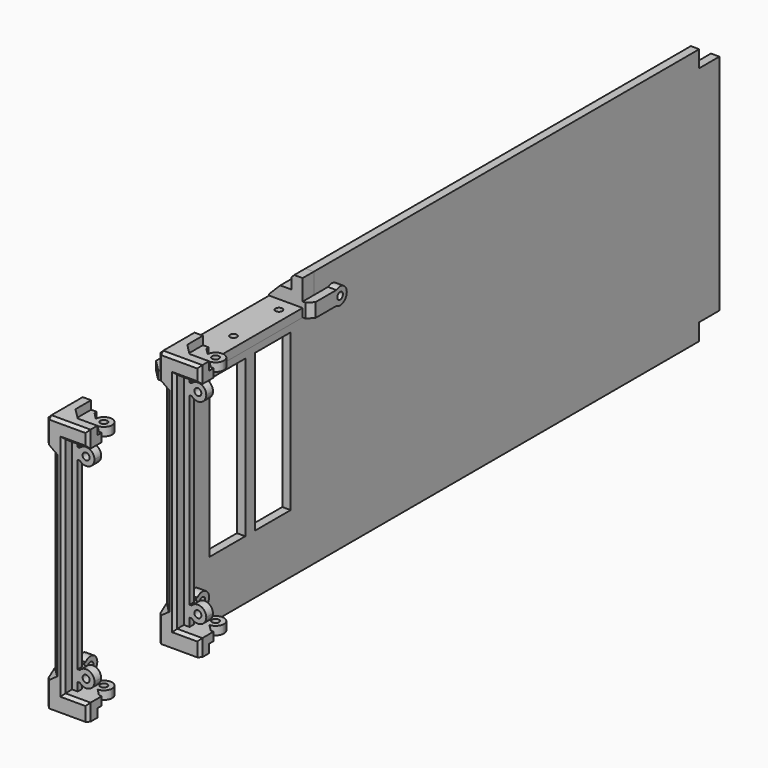
from build123d import *

# Parameters (mm, degrees)
F1_DEPTH     = 6
F2_W         = 2
F2_H         = 2
F3_DEPTH     = 5
F5_DEPTH     = 35
F7_DEPTH     = 3
F8_R         = 1.25
F9_DEPTH     = 3
F11_DEPTH    = 4
F13_DEPTH    = 3
F15_DEPTH    = 3
F17_SIZE     = 0.99999
F18_SIZE     = 2
F20_W        = 7.1945152003
F20_H        = 11.8572201729
F21_DEPTH    = 25
F23_W        = 10
F23_H        = 5
F24_DEPTH    = 4
F25_W        = 5
F25_H        = 4.5
F25_W_2      = 3
F25_W_3      = 7
F25_H_2      = 3
F26_DEPTH    = 8
F27_SIZE     = 4
F28_SIZE     = 3
F29_R        = 1.25
F30_DEPTH    = 3
F31_W        = 5
F31_H        = 5
F32_DEPTH    = 3
F33_SIZE     = 2
F34_T1_DEPTH = 3.071682988
F34_T3_DEPTH = 10.1433659759
F34_T5_DEPTH = 7.471682988
F36_DEPTH    = 3
F22_W        = 7.95
F22_H        = 56
F22_W_2      = 15.9
F37_DEPTH    = 25


# Not quite as in the source:
# - a fillet or chamfer that OpenCascade refuses, or shapes differently, is made with other operations: its cross-section is extruded or revolved along the edge and cut away or added
# - a fillet or chamfer is up to 0.001 mm smaller than in the source, because OpenCascade refuses the exact size
# - a feature names something its author has since deleted; it is built from what else it names


with BuildPart() as f1:
    # F0 (on Top) → F1 (new body)
    with BuildSketch(Plane.XY):
        Polygon((-29.7051688433, 8.7922193985), (-30.7051688433, 8.7922193985), (-30.7051688433, -6.2077806015), (-15.7051688433, -6.2077806015), (-15.7051688433, -5.2077806015), (-15.7051688433, -0.2077806015), (-24.7051688433, -0.2077806015), (-24.7051688433, 8.7922193985), align=None)
    extrude(amount=F1_DEPTH)

    # F2 (on face) → F3 (join)
    with BuildSketch(Plane.XY.offset(6)):
        with Locations((-23.7051688433, -1.2077806015)):
            Rectangle(F2_W, F2_H)
        Polygon((-26.7051688433, -0.2077806015), (-30.7051688433, -0.2077806015), (-30.7051688433, -5.2077806015), (-29.7051688433, -6.2077806015), (-24.7051688433, -6.2077806015), (-24.7051688433, -2.2077806015), (-24.7051688433, -0.2077806015), align=None)
        with Locations((-25.7051688433, 0.7922193985)):
            Rectangle(F2_W, F2_H)
    extrude(amount=F3_DEPTH)

    # F4 (on face) → F5 (join)
    with BuildSketch(Plane.XY.offset(11)):
        Polygon((-26.7051688433, -6.2077806015), (-24.7051688433, -6.2077806015), (-24.7051688433, -2.2077806015), (-22.7051688433, -2.2077806015), (-22.7051688433, -0.2077806015), (-24.7051688433, -0.2077806015), (-24.7051688433, 1.7922193985), (-26.7051688433, 1.7922193985), (-26.7051688433, -0.2077806015), (-30.7051688433, -0.2077806015), (-30.7051688433, -2.2077806015), align=None)
    extrude(amount=F5_DEPTH)

    # F6 (on face) → F7 (join)
    with BuildSketch(Plane.XZ.offset(2.2077806015)):
        with BuildLine():
            ThreePointArc((-21.9412368208, 13), (-22.5076859202, 12.0704662693), (-22.7051688433, 11))
            ThreePointArc((-22.7051688433, 11), (-22.5076859202, 9.9295337307), (-21.9412368208, 9))
            ThreePointArc((-21.9412368208, 9), (-18.634702574, 8.1974829231), (-16.7051688433, 11))
            ThreePointArc((-16.7051688433, 11), (-18.634702574, 13.8025170769), (-21.9412368208, 13))
        make_face()
        with BuildLine():
            ThreePointArc((-18.4551688433, 11), (-19.7051688433, 9.75), (-20.9551688433, 11))
            ThreePointArc((-20.9551688433, 11), (-19.7051688433, 12.25), (-18.4551688433, 11))
        make_face(mode=Mode.SUBTRACT)
        with BuildLine():
            Line((-22.7051688433, 13), (-22.7051688433, 11))
            ThreePointArc((-22.7051688433, 11), (-22.5076859202, 12.0704662693), (-21.9412368208, 13))
            Line((-21.9412368208, 13), (-22.7051688433, 13))
        make_face()
        with BuildLine():
            Line((-22.7051688433, 11), (-22.7051688433, 9))
            Line((-22.7051688433, 9), (-21.9412368208, 9))
            ThreePointArc((-21.9412368208, 9), (-22.5076859202, 9.9295337307), (-22.7051688433, 11))
        make_face()
    extrude(amount=-F7_DEPTH)

    # F8 (on face) → F9 (join)
    with BuildSketch(Plane(origin=(-26.7051688433, 0, 0), x_dir=(0, -1, 0), z_dir=(-1, 0, 0))):
        with BuildLine():
            Line((-2.556151421, 9), (-1.7922193985, 9))
            Line((-1.7922193985, 9), (-1.7922193985, 11))
            ThreePointArc((-1.7922193985, 11), (-1.9897023217, 9.9295337307), (-2.556151421, 9))
        make_face()
        with BuildLine():
            ThreePointArc((-2.556151421, 13), (-1.9897023217, 12.0704662693), (-1.7922193985, 11))
            Line((-1.7922193985, 11), (-1.7922193985, 13))
            Line((-1.7922193985, 13), (-2.556151421, 13))
        make_face()
        with BuildLine():
            ThreePointArc((-2.556151421, 9), (-1.9897023217, 9.9295337307), (-1.7922193985, 11))
            ThreePointArc((-1.7922193985, 11), (-1.9897023217, 12.0704662693), (-2.556151421, 13))
            ThreePointArc((-2.556151421, 13), (-7.7922193985, 11), (-2.556151421, 9))
        make_face()
        with Locations((-4.7922193985, 11)):
            Circle(F8_R, mode=Mode.SUBTRACT)
    extrude(amount=-F9_DEPTH)

    # F10 (on face) → F11 (join)
    with BuildSketch(Plane.XY.offset(13)):
        Polygon((-22.7051688433, 0.7922193985), (-23.7051688433, 1.7922193985), (-24.7051688433, 1.7922193985), (-24.7051688433, -0.2077806015), (-22.7051688433, -0.2077806015), align=None)
    extrude(amount=-F11_DEPTH)

    # F12 (on face) → F13 (cut)
    with BuildSketch(Plane(origin=(0, 0, 0), x_dir=(1, 0, 0), z_dir=(0, 0, -1))):
        Polygon((-24.7051688433, -8.7922193985), (-24.7051688433, 0.2077806015), (-26.7051688433, -1.7922193985), (-26.7051688433, -8.7922193985), align=None)
        Polygon((-24.7051688433, 0.2077806015), (-15.7051688433, 0.2077806015), (-15.7051688433, 2.2077806015), (-22.7051688433, 2.2077806015), align=None)
    extrude(amount=-F13_DEPTH, mode=Mode.SUBTRACT)

    # F14 (on face) → F15 (join)
    with BuildSketch(Plane(origin=(0, 0, 3), x_dir=(1, 0, 0), z_dir=(0, 0, -1))):
        with BuildLine():
            Line((-16.7051688433, 0.2077806015), (-24.7051688433, 0.2077806015))
            Line((-24.7051688433, 0.2077806015), (-24.7051688433, -7.7922193985))
            Line((-24.7051688433, -7.7922193985), (-22.2863076734, -5.3733582286))
            ThreePointArc((-22.2863076734, -5.3733582286), (-21.4122756245, -3.0851126174), (-19.1240300132, -2.2110805685))
            Line((-19.1240300132, -2.2110805685), (-16.7051688433, 0.2077806015))
        make_face()
        with BuildLine():
            ThreePointArc((-19.1240300132, -2.2110805685), (-21.4122756245, -3.0851126174), (-22.2863076734, -5.3733582286))
            Line((-22.2863076734, -5.3733582286), (-20.7051688433, -3.7922193985))
            Line((-20.7051688433, -3.7922193985), (-19.1240300132, -2.2110805685))
        make_face()
        with BuildLine():
            Line((-20.7051688433, -3.7922193985), (-22.2863076734, -5.3733582286))
            ThreePointArc((-22.2863076734, -5.3733582286), (-19.2074603031, -8.2052708339), (-16.2909552809, -5.2064329609))
            ThreePointArc((-16.2909552809, -5.2064329609), (-17.1114168202, -3.1449742302), (-19.1240300132, -2.2110805685))
            Line((-19.1240300132, -2.2110805685), (-20.7051688433, -3.7922193985))
        make_face()
        with BuildLine():
            ThreePointArc((-18.0409552809, -5.2064329609), (-19.7693095714, -6.3612823766), (-20.1748387574, -4.3225494844))
            ThreePointArc((-20.1748387574, -4.3225494844), (-18.8126009904, -4.0515835453), (-18.0409552809, -5.2064329609))
        make_face(mode=Mode.SUBTRACT)
    extrude(amount=-F15_DEPTH)

    # F16: F1 across face


with BuildPart() as f1_1:
    add(f1.part)
    add(f1.part.mirror(Plane(origin=(-26.6681318062, -2.1707435644, 46), x_dir=(1, 0, 0), z_dir=(0, 0, 1))))

    # F17 (size 1 in the source; OpenCascade refuses exactly that, so slightly less here)
    f17_edges = [f1_1.edges().sort_by_distance(p)[0] for p in [
        (-24.705169, -6.207781, 46),
        (-20.205169, -6.207781, 6),
        (-30.705169, 4.292219, 6),
        (-30.705169, -0.207781, 46),
        (-30.705169, 4.292219, 86),
        (-20.205169, -6.207781, 86),
        (-15.705169, -6.207781, 89),
        (-30.705169, 8.792219, 89),
        (-23.205169, -6.207781, 92),
        (-30.705169, -6.207781, 89),
        (-30.705169, 1.292219, 92),
        (-30.705169, 8.792219, 3),
        (-30.705169, -6.207781, 3),
        (-15.705169, -6.207781, 3),
    ]]
    chamfer(f17_edges, length=F17_SIZE)

    # F18
    f18_edges = [f1_1.edges().sort_by_distance(p)[0] for p in [
        (-30.205169, -5.707781, 11),
        (-30.205169, -5.707781, 81),
    ]]
    chamfer(f18_edges, length=F18_SIZE)


with BuildPart() as f19_1:
    # F19: copy of F1
    add(f1_1.part.moved(Location((0, 50, 0))))

    # F20 (on face) → F21 (cut)
    with BuildSketch(Plane(origin=(-26.7051688433, 0, 0), x_dir=(0, -1, 0), z_dir=(-1, 0, 0))):
        with Locations((-55.3894769987, 80.0713899136)):
            Rectangle(F20_W, F20_H)
    extrude(amount=-F21_DEPTH, mode=Mode.SUBTRACT)

    # F23 (on face) → F24 (join)
    with BuildSketch(Plane(origin=(-26.7051688433, 0, 0), x_dir=(0, -1, 0), z_dir=(-1, 0, 0))):
        Polygon((-108.3922193985, 79.6), (-98.3922193985, 79.6), (-98.3922193985, 82.6), (-103.3922193985, 82.6), (-103.3922193985, 89), (-103.3922193985, 92), (-108.3922193985, 92), align=None)
        Polygon((-98.3922193985, 82.6), (-98.3922193985, 79.6), (-49.7922193985, 79.6), (-48.7922193985, 79.6), (-48.7922193985, 82.6), (-58.7922193985, 82.6), (-78.0922193985, 82.6), align=None)
        with Locations((-53.7922193985, 85.1)):
            Rectangle(F23_W, F23_H)
    extrude(amount=F24_DEPTH)

    # F25 (on face) → F26 (join)
    with BuildSketch(Plane(origin=(-30.7051688433, 0, 0), x_dir=(0, -1, 0), z_dir=(-1, 0, 0))):
        with Locations((-105.8922193985, 84.85)):
            Rectangle(F25_W, F25_H)
        Polygon((-58.7922193985, 82.6), (-103.3922193985, 82.6), (-108.3922193985, 82.6), (-108.3922193985, 79.6), (-55.7922193985, 79.6), (-55.7922193985, 82.6), align=None)
        with Locations((-57.2922193985, 84.85)):
            Rectangle(F25_W_2, F25_H)
        with Locations((-52.2922193985, 81.1)):
            Rectangle(F25_W_3, F25_H_2)
    extrude(amount=F26_DEPTH)

    # F27
    f27_edges = [f19_1.edges().sort_by_distance(p)[0] for p in [
        (-38.705169, 48.792219, 81.1),
        (-38.705169, 57.292219, 87.1),
        (-38.705169, 105.892219, 87.1),
    ]]
    chamfer(f27_edges, length=F27_SIZE)

    # F28
    f28_edges = [f19_1.edges().sort_by_distance(p)[0] for p in [
        (-38.705169, 108.392219, 81.35),
    ]]
    chamfer(f28_edges, length=F28_SIZE)

    # F29 (on face) → F30 (cut)
    with BuildSketch(Plane.XY.offset(82.6)):
        with Locations((-31.2051688433, 98.3922193985)):
            Circle(F29_R)
        with Locations((-31.2051688433, 78.0922193985)):
            Circle(F29_R)
    extrude(amount=-F30_DEPTH, mode=Mode.SUBTRACT)

    # F31 (on face) → F32 (join)
    with BuildSketch(Plane.YZ.offset(-26.7051688433)):
        Polygon((108.3922193985, 84.6), (108.3922193985, 79.6), (113.3922193985, 79.6), (113.3922193985, 82.1), (113.3922193985, 84.6), align=None)
        with Locations((105.8922193985, 82.1)):
            Rectangle(F31_W, F31_H)
        with BuildLine():
            Line((113.3922193985, 82.1), (113.3922193985, 79.6))
            Line((113.3922193985, 79.6), (114.7339070034, 79.6))
            ThreePointArc((114.7339070034, 79.6), (113.7488373617, 80.6813628345), (113.3922193985, 82.1))
        make_face()
        with BuildLine():
            Line((113.3922193985, 84.6), (113.3922193985, 82.1))
            ThreePointArc((113.3922193985, 82.1), (113.7488373617, 83.5186371655), (114.7339070034, 84.6))
            Line((114.7339070034, 84.6), (113.3922193985, 84.6))
        make_face()
        with BuildLine():
            ThreePointArc((114.7339070034, 84.6), (113.7488373617, 83.5186371655), (113.3922193985, 82.1))
            ThreePointArc((113.3922193985, 82.1), (113.7488373617, 80.6813628345), (114.7339070034, 79.6))
            ThreePointArc((114.7339070034, 79.6), (117.810856564, 79.4566179631), (119.3922193985, 82.1))
            ThreePointArc((119.3922193985, 82.1), (117.810856564, 84.7433820369), (114.7339070034, 84.6))
        make_face()
        with BuildLine():
            ThreePointArc((117.6422193985, 82.1), (116.3922193985, 80.85), (115.1422193985, 82.1))
            ThreePointArc((115.1422193985, 82.1), (116.3922193985, 83.35), (117.6422193985, 82.1))
        make_face(mode=Mode.SUBTRACT)
    extrude(amount=F32_DEPTH)

    # F33
    f33_edges = [f19_1.edges().sort_by_distance(p)[0] for p in [
        (-23.705169, 103.392219, 82.1),
    ]]
    chamfer(f33_edges, length=F33_SIZE)

    # F34: chamfer of 1 on 3 edges, made by hand

    # F34_s2 → F34_t1 (cut)
    with BuildSketch(Plane.XY.offset(87.1)):
        Polygon((-30.7051688433, 57.7922193985), (-29.7051688433, 58.7922193985), (-30.7051688433, 58.7922193985), align=None)
    extrude(amount=F34_T1_DEPTH, mode=Mode.SUBTRACT)

    # F34_s4 → F34_t3 (cut)
    with BuildSketch(Plane.XZ.offset(-110.9639023865)):
        Polygon((-29.7051688433, 92), (-30.7051688433, 91), (-30.7051688433, 92), align=None)
    extrude(amount=F34_T3_DEPTH, mode=Mode.SUBTRACT)

    # F34_s6 → F34_t5 (cut)
    with BuildSketch(Plane.XY.offset(87.1)):
        Polygon((-30.7051688433, 107.3922193985), (-29.7051688433, 108.3922193985), (-30.7051688433, 108.3922193985), align=None)
    extrude(amount=F34_T5_DEPTH, mode=Mode.SUBTRACT)


with BuildPart() as f36:
    # F35 (on face) → F36 (new body)
    with BuildSketch(Plane(origin=(-26.7051688433, 0, 0), x_dir=(0, -1, 0), z_dir=(-1, 0, 0))):
        Polygon((-58.7922193985, 6), (-49.7922193985, 6), (-49.7922193985, 79.6), (-108.3922193985, 79.6), (-108.3922193985, 92), (-280.7922193985, 92), (-280.7922193985, 86), (-289.7922193985, 86), (-289.7922193985, 6), (-280.7922193985, 6), (-280.7922193985, 0), (-58.7922193985, 0), align=None)
    extrude(amount=F36_DEPTH)

    # F22 (on face) → F37 (cut)
    with BuildSketch(Plane(origin=(-26.7051688433, 0, 0), x_dir=(0, -1, 0), z_dir=(-1, 0, 0))):
        with Locations((-86.1172193985, 49.1)):
            Rectangle(F22_W, F22_H)
        with Locations((-94.0672193985, 49.1)):
            Rectangle(F22_W, F22_H)
        with Locations((-69.7922193985, 49.1)):
            Rectangle(F22_W_2, F22_H)
    extrude(amount=F37_DEPTH, mode=Mode.SUBTRACT)


solid = Compound([f1_1.part, f19_1.part, f36.part])
